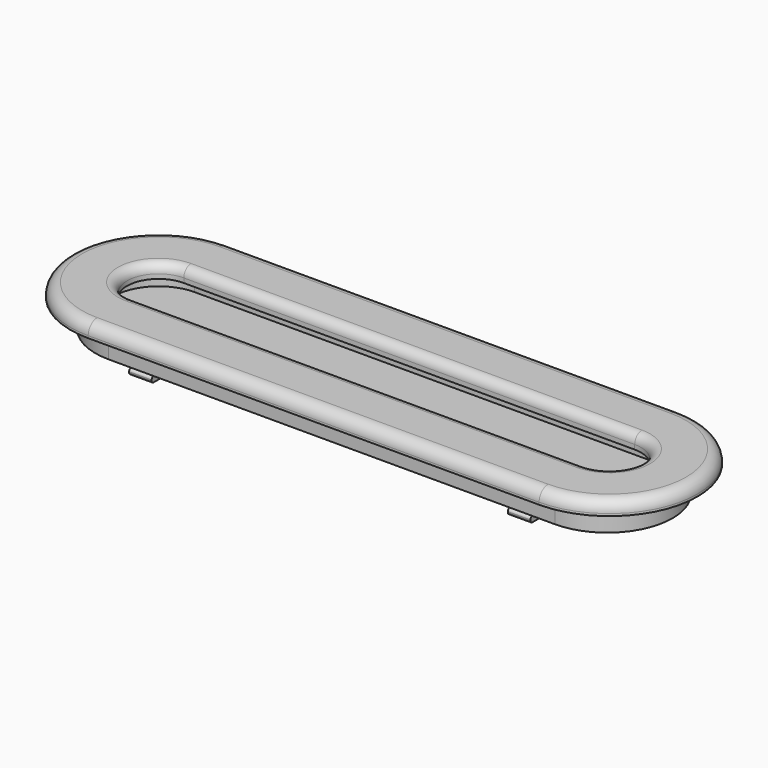
from build123d import *

# Parameters (mm, degrees)
F1_DEPTH  = 6
F3_DEPTH  = 3
F4_R      = 2.5
F5_W      = 5
F5_H      = 30.1
F6_DEPTH  = 1.25
F8_DEPTH  = 6
F10_DEPTH = 3
F11_R     = 2
F12_R     = 0.54999


# Not quite as in the source:
# - a fillet or chamfer is up to 0.001 mm smaller than in the source, because OpenCascade refuses the exact size


with BuildPart() as f1:
    # F0 (on Top) → F1 (new body)
    with BuildSketch(Plane.XY):
        with BuildLine():
            Line((49.5, 14.5), (-49.5, 14.5))
            ThreePointArc((-49.5, 14.5), (-64, 0), (-49.5, -14.5))
            Line((-49.5, -14.5), (49.5, -14.5))
            ThreePointArc((49.5, -14.5), (64, 0), (49.5, 14.5))
        make_face()
    extrude(amount=F1_DEPTH)

    # F2 (on face) → F3 (join)
    with BuildSketch(Plane.XY.offset(6)):
        with BuildLine():
            Line((50, 19.5), (-50, 19.5))
            ThreePointArc((-50, 19.5), (-69.5, 0), (-50, -19.5))
            Line((-50, -19.5), (50, -19.5))
            ThreePointArc((50, -19.5), (69.5, 0), (50, 19.5))
        make_face()
    extrude(amount=F3_DEPTH)

    # F4
    f4_edges = [f1.edges().sort_by_distance(p)[0] for p in [
        (0, -19.5, 9),
    ]]
    fillet(f4_edges, radius=F4_R)

    # F5 (on face) → F6 (join)
    with BuildSketch(Plane(origin=(0, 0, 0), x_dir=(1, 0, 0), z_dir=(0, 0, -1))):
        with Locations((-42, 0)):
            Rectangle(F5_W, F5_H)
        with Locations((42, 0)):
            Rectangle(F5_W, F5_H)
    extrude(amount=F6_DEPTH)

    # F7 (on face) → F8 (cut)
    with BuildSketch(Plane.XY.offset(9)):
        with BuildLine():
            Line((50, 10), (-50, 10))
            ThreePointArc((-50, 10), (-60, 0), (-50, -10))
            Line((-50, -10), (50, -10))
            ThreePointArc((50, -10), (60, 0), (50, 10))
        make_face()
    extrude(amount=-F8_DEPTH, mode=Mode.SUBTRACT)

    # F9 (on face) → F10 (join)
    with BuildSketch(Plane.XY.offset(9)):
        with BuildLine():
            Line((50, 10), (-50, 10))
            ThreePointArc((-50, 10), (-60, 0), (-50, -10))
            Line((-50, -10), (50, -10))
            ThreePointArc((50, -10), (60, 0), (50, 10))
        make_face()
        with BuildLine():
            ThreePointArc((50, 7), (57, 0), (50, -7))
            Line((50, -7), (-50, -7))
            ThreePointArc((-50, -7), (-57, 0), (-50, 7))
            Line((-50, 7), (50, 7))
        make_face(mode=Mode.SUBTRACT)
    extrude(amount=-F10_DEPTH)

    # F11
    f11_edges = [f1.edges().sort_by_distance(p)[0] for p in [
        (0, 7, 9),
    ]]
    fillet(f11_edges, radius=F11_R)

    # F12 (radius 0.55 in the source; OpenCascade refuses exactly that, so slightly less here)
    f12_edges = [f1.edges().sort_by_distance(p)[0] for p in [
        (-42, -15.05, 0),
        (-42, -15.05, -1.25),
        (42, -15.05, -1.25),
        (42, -15.05, 0),
        (-42, 15.05, -1.25),
        (-42, 15.05, 0),
        (42, 15.05, 0),
        (42, 15.05, -1.25),
    ]]
    fillet(f12_edges, radius=F12_R)


solid = f1.part
